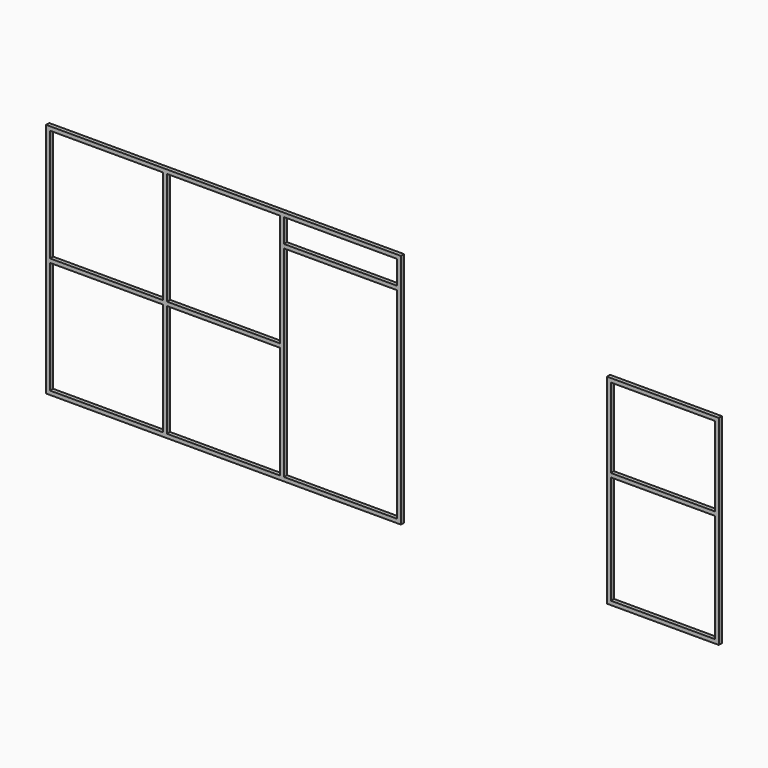
from build123d import *

# Parameters (mm, degrees)
F0_W     = 3000
F0_H     = 2000
F0_W_2   = 956
F0_H_2   = 950.5
F0_H_3   = 200
F1_DEPTH = 33
F2_W     = 946
F2_H     = 1690
F2_W_2   = 880
F2_H_2   = 33
F3_DEPTH = 33


# Not quite as in the source:
# - a feature names something its author has since deleted; it is built from what else it names


with BuildPart() as f1:
    # F0 (on Front) → F1 (new body)
    with BuildSketch(Plane.XZ):
        with Locations((1500, 1000)):
            Rectangle(F0_W, F0_H)
        with Locations((511, 508.25)):
            Rectangle(F0_W_2, F0_H_2, mode=Mode.SUBTRACT)
        with Locations((1500, 508.25)):
            Rectangle(F0_W_2, F0_H_2, mode=Mode.SUBTRACT)
        Polygon((2967, 33), (2011, 33), (2011, 1734), (2967, 1734), (2967, 1016.5), (2967, 983.5), align=None, mode=Mode.SUBTRACT)
        with Locations((511, 1491.75)):
            Rectangle(F0_W_2, F0_H_2, mode=Mode.SUBTRACT)
        with Locations((1500, 1491.75)):
            Rectangle(F0_W_2, F0_H_2, mode=Mode.SUBTRACT)
        with Locations((2489, 1867)):
            Rectangle(F0_W_2, F0_H_3, mode=Mode.SUBTRACT)
    extrude(amount=F1_DEPTH)


with BuildPart() as f3:
    # F2 (on face) → F3 (new body)
    with BuildSketch(Plane.XZ.offset(33)):
        with Locations((5240.176655467, 845)):
            Rectangle(F2_W, F2_H)
        Polygon((4800.176655467, 983.5), (4800.176655467, 1657), (5680.176655467, 1657), (5680.176655467, 983.5), (5680.176655467, 950.5), (5680.176655467, 33), (4800.176655467, 33), (4800.176655467, 950.5), align=None, mode=Mode.SUBTRACT)
        with Locations((5240.176655467, 967)):
            Rectangle(F2_W_2, F2_H_2)
    extrude(amount=F3_DEPTH)


solid = Compound([f1.part, f3.part])
